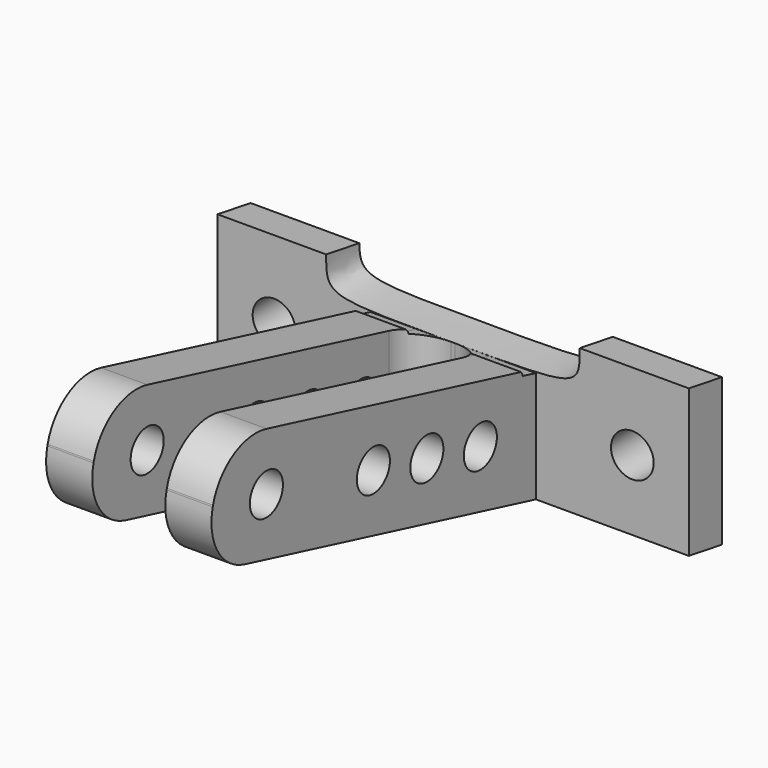
from build123d import *

# Parameters (mm, degrees)
F0_R          = 1.55
F1_DEPTH      = 3
F2_SIZE2      = 2.99999
F2_SIZE       = 0.49999
F2_2_SIZE2    = 2.99999
F2_2_SIZE     = 0.49999
F4_DEPTH      = 6
F5_DEPTH      = 6
F6_R          = 1.5
F7_DEPTH      = 25
F9_W          = 5.3
F9_H          = 30.2732266598
F10_DEPTH     = 25
F11_R         = 4
F12_T4_DEPTH  = 20.5670004785
F12_T10_DEPTH = 20.5670004785
F12_T16_DEPTH = 20.5670004785
F12_T22_DEPTH = 20.5670004785
F13_SIZE      = 0.2


# Not quite as in the source:
# - a fillet or chamfer that OpenCascade refuses, or shapes differently, is made with other operations: its cross-section is extruded or revolved along the edge and cut away or added
# - a fillet or chamfer is up to 0.001 mm smaller than in the source, because OpenCascade refuses the exact size
# - ends of sketch curves that miss each other by under 0.0002 mm in the source are joined


with BuildPart() as f1:
    # F0 (on Front) → F1 (new body)
    with BuildSketch(Plane.XZ):
        with BuildLine():
            Line((-17.1, 5.6), (-17.1, -5.6))
            Line((-17.1, -5.6), (17.1, -5.6))
            Line((17.1, -5.6), (17.1, 5.6))
            Line((17.1, 5.6), (9.1844569534, 5.6))
            add(Edge.make_bspline(
                [(9.1844569534, 5.6), (9.1844569534, 2.9670004785), (9.1844569534, 2.9670004785), (-0.0155430466, 2.9670004785)],
                knots=[0, 0, 0, 0, 9.5693619495, 9.5693619495, 9.5693619495, 9.5693619495], degree=3))
            add(Edge.make_bspline(
                [(-9.2155430466, 5.6), (-9.2155430466, 2.9670004785), (-9.2155430466, 2.9670004785), (-0.0155430466, 2.9670004785)],
                knots=[0, 0, 0, 0, 9.5693618638, 9.5693618638, 9.5693618638, 9.5693618638], degree=3))
            Line((-9.2155430466, 5.6), (-17.1, 5.6))
        make_face()
        with Locations((-13, 0)):
            Circle(F0_R, mode=Mode.SUBTRACT)
        with Locations((13, 0)):
            Circle(F0_R, mode=Mode.SUBTRACT)
    extrude(amount=F1_DEPTH)

    # F2 (size 0.5 and 3 in the source; OpenCascade refuses exactly that, so slightly less here)
    f2_edges = [f1.edges().sort_by_distance(p)[0] for p in [
        (-13.157772, 0, 5.6),
        (13.142228, 0, 5.6),
    ]]
    f2_side = f1.faces().sort_by_distance((0.002222, 0, -0.619959))[0]
    chamfer(f2_edges, length=F2_SIZE, length2=F2_SIZE2, reference=f2_side)

    # F2#2 (size 0.5 and 3 in the source; OpenCascade refuses exactly that, so slightly less here)
    f2_2_edges = [f1.edges().sort_by_distance(p)[0] for p in [
        (0, -3, -5.6),
    ]]
    f2_2_side = f1.faces().sort_by_distance((0.002222, -3, -0.619959))[0]
    chamfer(f2_2_edges, length=F2_2_SIZE, length2=F2_2_SIZE2, reference=f2_2_side)

    # F3 (on Right) → F4 (join)
    with BuildSketch(Plane.YZ):
        Polygon((-33.2732266598, 2.4479631427), (-3, -5.1), (-3, 2.9670004785), (-4.2113326633, 3.2690196322), (-4.1453789697, 3.5335454488), (-31.3136593055, 10.3073585255), align=None)
    extrude(amount=F4_DEPTH)

    # F5 (add): a face of the model
    f5_faces = [f1.faces().sort_by_distance(p)[0] for p in [
        (0, -17.6712487641, 2.6798726591),
    ]]
    extrude(f5_faces, amount=F5_DEPTH)

    # F6 (on face) → F7 (cut)
    with BuildSketch(Plane.YZ.offset(6)):
        with Locations((-27.4419643513, 5.1680513561)):
            Circle(F6_R)
        with Locations((-17.7390070885, 2.7488324001)):
            Circle(F6_R)
        with Locations((-12.8875284571, 1.5392229221)):
            Circle(F6_R)
        with Locations((-8.0360498257, 0.3296134441)):
            Circle(F6_R)
    extrude(amount=-F7_DEPTH, mode=Mode.SUBTRACT)

    # F9 (on face) → F10 (cut)
    with BuildSketch(Plane(origin=(0, 0, -5.6), x_dir=(1, 0, 0), z_dir=(0, 0, -1))):
        with Locations((0, 18.1366133299)):
            Rectangle(F9_W, F9_H)
    extrude(amount=-F10_DEPTH, mode=Mode.SUBTRACT)

    # F11
    f11_edges = [f1.edges().sort_by_distance(p)[0] for p in [
        (-4.325, -33.273227, 2.447963),
        (4.325, -33.273227, 2.447963),
        (-4.325, -31.313659, 10.307359),
        (4.325, -31.313659, 10.307359),
    ]]
    fillet(f11_edges, radius=F11_R)

    # F12: fillet of radius 2.5 on 2 edges, made by hand


with BuildPart() as f12_tool2:
    # F12_s3 → F12_t4 (new body)
    with BuildSketch(Plane.XY.offset(-11.35)):
        with BuildLine():
            ThreePointArc((-0.15, -3), (-1.917766953, -3.732233047), (-2.65, -5.5))
            Line((-2.65, -5.5), (-2.65, -3))
            Line((-2.65, -3), (-0.15, -3))
        make_face()
    extrude(amount=F12_T4_DEPTH)

    split(bisect_by=Plane(origin=(0, 0.520882565, 2.0891458603), x_dir=(1, 0, 0), z_dir=(0, -0.2419218956, -0.9702957263)), keep=Keep.TOP)

    split(bisect_by=Plane(origin=(0, -1.3727310958, -5.505723706), x_dir=(1, 0, 0), z_dir=(0, 0.2419218956, 0.9702957263)), keep=Keep.TOP)


with BuildPart() as f1_1:
    add(f1.part)

    # F12_t1: union F12_tool2
    add(f12_tool2.part)


with BuildPart() as f12_tool8:
    # F12_s9 → F12_t10 (new body)
    with BuildSketch(Plane.XY.offset(-11.35)):
        with BuildLine():
            ThreePointArc((-0.15, -3), (-1.917766953, -3.732233047), (-2.65, -5.5))
            Line((-2.65, -5.5), (-2.65, -3))
            Line((-2.65, -3), (-0.15, -3))
        make_face()
    extrude(amount=F12_T10_DEPTH)

    split(bisect_by=Plane(origin=(0, -4.7322152283, 1.1798737719), x_dir=(1, 0, 0), z_dir=(0, -0.9702957263, 0.2419218956)), keep=Keep.TOP)

    split(bisect_by=Plane(origin=(0, 0.5868362585, 2.3536716769), x_dir=(1, 0, 0), z_dir=(0, -0.2419218956, -0.9702957263)), keep=Keep.TOP)


with BuildPart() as f1_2:
    add(f1_1.part)

    # F12_t7: union F12_tool8
    add(f12_tool8.part)


with BuildPart() as f12_tool14:
    # F12_s15 → F12_t16 (new body)
    with BuildSketch(Plane.XY.offset(-11.35)):
        with BuildLine():
            ThreePointArc((0.15, -3), (1.917766953, -3.732233047), (2.65, -5.5))
            Line((2.65, -5.5), (2.65, -3))
            Line((2.65, -3), (0.15, -3))
        make_face()
    extrude(amount=F12_T16_DEPTH)

    split(bisect_by=Plane(origin=(0, -1.3727310958, -5.505723706), x_dir=(1, 0, 0), z_dir=(0, 0.2419218956, 0.9702957263)), keep=Keep.TOP)

    split(bisect_by=Plane(origin=(0, 0.520882565, 2.0891458603), x_dir=(1, 0, 0), z_dir=(0, -0.2419218956, -0.9702957263)), keep=Keep.TOP)


with BuildPart() as f1_3:
    add(f1_2.part)

    # F12_t13: union F12_tool14
    add(f12_tool14.part)


with BuildPart() as f12_tool20:
    # F12_s21 → F12_t22 (new body)
    with BuildSketch(Plane.XY.offset(-11.35)):
        with BuildLine():
            ThreePointArc((0.15, -3), (1.917766953, -3.732233047), (2.65, -5.5))
            Line((2.65, -5.5), (2.65, -3))
            Line((2.65, -3), (0.15, -3))
        make_face()
    extrude(amount=F12_T22_DEPTH)

    split(bisect_by=Plane(origin=(0, -4.7322152283, 1.1798737719), x_dir=(1, 0, 0), z_dir=(0, -0.9702957263, 0.2419218956)), keep=Keep.TOP)

    split(bisect_by=Plane(origin=(0, 0.5868362585, 2.3536716769), x_dir=(1, 0, 0), z_dir=(0, -0.2419218956, -0.9702957263)), keep=Keep.TOP)


with BuildPart() as f1_4:
    add(f1_3.part)

    # F12_t19: union F12_tool20
    add(f12_tool20.part)

    # F13
    f13_edges = [f1_4.edges().sort_by_distance(p)[0] for p in [
        (4.125595, -4.145379, 3.533545),
        (-4.125595, -4.145379, 3.533545),
    ]]
    chamfer(f13_edges, length=F13_SIZE)


solid = f1_4.part
